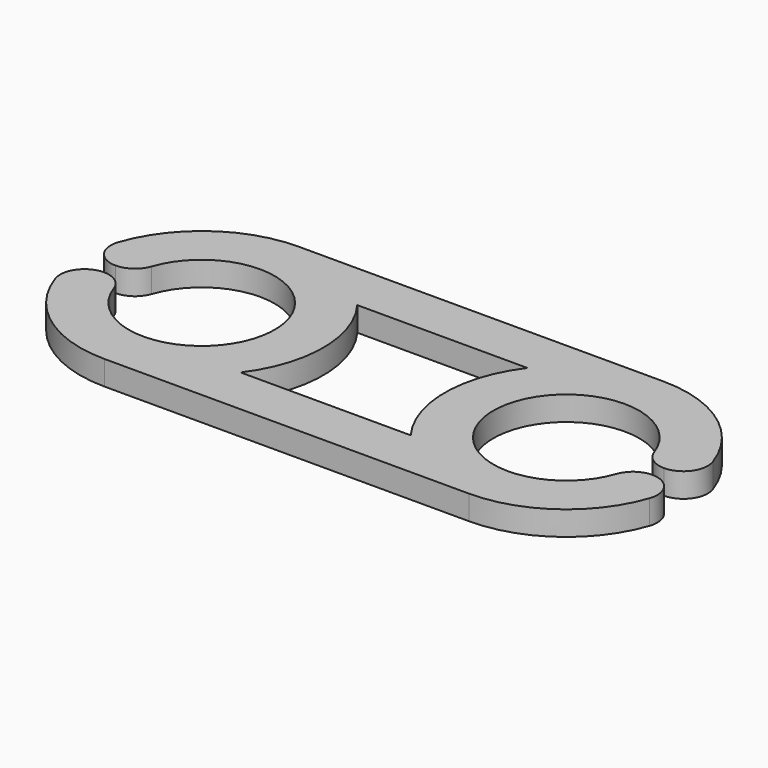
from build123d import *

# Parameters (mm, degrees)
F1_DEPTH = 1.27
F2_R     = 7.62
F3_DEPTH = 25.4
F5_W     = 12.5357808316
F5_H     = 1.524
F6_DEPTH = 25.4
F7_R     = 2.53999


# Not quite as in the source:
# - a fillet or chamfer is up to 0.001 mm smaller than in the source, because OpenCascade refuses the exact size


with BuildPart() as f1:
    # F0 (on Top) → F1 (new body, symmetric)
    with BuildSketch(Plane.XY):
        with BuildLine():
            Line((19.05, 12.7), (-19.05, 12.7))
            ThreePointArc((-19.05, 12.7), (-31.75, 0), (-19.05, -12.7))
            Line((-19.05, -12.7), (19.05, -12.7))
            ThreePointArc((19.05, -12.7), (31.75, 0), (19.05, 12.7))
        make_face()
    extrude(amount=F1_DEPTH, both=True)

    # F2 (on face) → F3 (cut)
    with BuildSketch(Plane.XY.offset(1.27)):
        with Locations((-19.05, 0)):
            Circle(F2_R)
        with Locations((19.05, 0)):
            Circle(F2_R)
        with BuildLine():
            Line((8.89, 7.62), (-8.89, 7.62))
            ThreePointArc((-8.89, 7.62), (-6.35, 0), (-8.89, -7.62))
            Line((-8.89, -7.62), (8.89, -7.62))
            ThreePointArc((8.89, -7.62), (6.35, 0), (8.89, 7.62))
        make_face()
    extrude(amount=-F3_DEPTH, mode=Mode.SUBTRACT)

    # F5 (on face) → F6 (cut)
    with BuildSketch(Plane.XY.offset(1.27)):
        with Locations((-25.4821095842, 0)):
            Rectangle(F5_W, F5_H)
        with Locations((25.4821095842, 0)):
            Rectangle(F5_W, F5_H)
    extrude(amount=-F6_DEPTH, mode=Mode.SUBTRACT)

    # F7 (radius 2.54 in the source; OpenCascade refuses exactly that, so slightly less here)
    f7_edges = [f1.edges().sort_by_distance(p)[0] for p in [
        (26.631804, 0.762, 0),
        (26.631804, -0.762, 0),
        (-26.631804, 0.762, 0),
        (-26.631804, -0.762, 0),
        (-31.727119, -0.762, 0),
        (-31.727119, 0.762, 0),
        (31.727119, 0.762, 0),
        (31.727119, -0.762, 0),
    ]]
    fillet(f7_edges, radius=F7_R)


solid = f1.part
